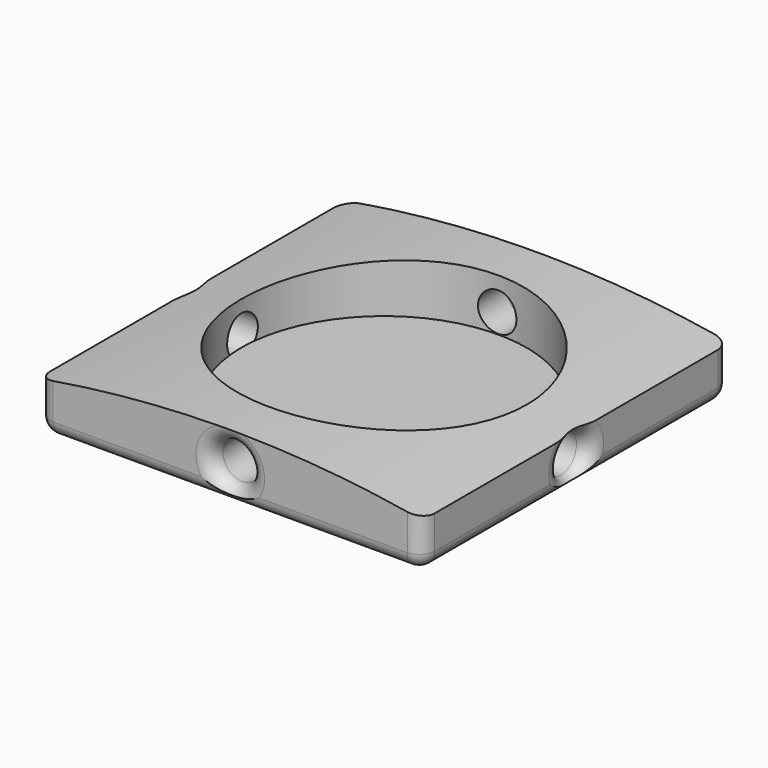
from build123d import *

# Parameters (mm, degrees)
F0_R         = 2.54
F1_DEPTH     = 25.4
F2_R         = 2.5365962647
F3_DEPTH     = 60.706
F4_R         = 18.8716899986
F5_DEPTH     = 14.478
F6_DEPTH     = 1.778
F7_T1_DEPTH  = 46.7340686292
F7_T3_DEPTH  = 46.7340686292
F7_T5_DEPTH  = 9.4612519522
F7_S9_W      = 2.2367022539
F7_S9_H      = 2.2367022539
F7_T10_DEPTH = 2.236702254
F7_S15_W     = 2.2367022539
F7_S15_H     = 2.2367022539
F7_T16_DEPTH = 2.236702254
F7_S21_W     = 2.2367022539
F7_S21_H     = 2.2367022539
F7_T22_DEPTH = 2.236702254
F7_S27_W     = 2.2367022539
F7_S27_H     = 2.2367022539
F7_T28_DEPTH = 2.236702254


# Not quite as in the source:
# - a fillet or chamfer that OpenCascade refuses, or shapes differently, is made with other operations: its cross-section is extruded or revolved along the edge and cut away or added


with BuildPart() as f1:
    # F0 (on Front) → F1 (new body, symmetric)
    with BuildSketch(Plane.XZ):
        with BuildLine():
            Line((25.4, 14.5918969065), (25.4, 21.0037002322))
            ThreePointArc((25.4, 21.0037002322), (0, 23.2693725585), (-25.4, 21.0037002322))
            Line((-25.4, 21.0037002322), (-25.4, 14.5918969065))
            Line((-25.4, 14.5918969065), (25.4, 14.5918969065))
        make_face()
        with Locations((0, 18.9952347428)):
            Circle(F0_R, mode=Mode.SUBTRACT)
    extrude(amount=F1_DEPTH, both=True)

    # F2 (on face) → F3 (cut)
    with BuildSketch(Plane.YZ.offset(25.4)):
        with Locations((0, 17.843645066)):
            Circle(F2_R)
    extrude(amount=-F3_DEPTH, mode=Mode.SUBTRACT)

    # F4 (on face) → F5 (cut)
    with BuildSketch(Plane(origin=(0, 0, 14.5918969065), x_dir=(1, 0, 0), z_dir=(0, 0, -1))):
        Circle(F4_R)
    extrude(amount=-F5_DEPTH, mode=Mode.SUBTRACT)

    # F4 (on face) → F6 (join)
    with BuildSketch(Plane(origin=(0, 0, 14.5918969065), x_dir=(1, 0, 0), z_dir=(0, 0, -1))):
        Circle(F4_R)
    extrude(amount=-F6_DEPTH)

    # F7: fillet of radius 2.032 on 12 edges, made by hand

    # F7_s2 → F7_t1 (cut)
    with BuildSketch(Plane.XZ.offset(-23.3670343146)):
        with BuildLine():
            ThreePointArc((-25.4004, 16.6248625919), (-24.8048409794, 15.1870559271), (-23.3670343146, 14.5914969065))
            Line((-23.3670343146, 14.5914969065), (-23.3670343146, 14.388160338))
            ThreePointArc((-23.3670343146, 14.388160338), (-24.3835171573, 14.388560338), (-25.4, 14.388560338))
            Line((-25.4, 14.388560338), (-25.6033365685, 14.5918969065))
            ThreePointArc((-25.6033365685, 14.5918969065), (-25.6033365685, 15.6083797492), (-25.6037365685, 16.6248625919))
            Line((-25.6037365685, 16.6248625919), (-25.4004, 16.6248625919))
        make_face()
        with BuildLine():
            ThreePointArc((25.4004, 16.6248625919), (24.8048409794, 15.1870559271), (23.3670343146, 14.5914969065))
            Line((23.3670343146, 14.5914969065), (23.3670343146, 14.388160338))
            ThreePointArc((23.3670343146, 14.388160338), (24.3835171573, 14.388560338), (25.4, 14.388560338))
            Line((25.4, 14.388560338), (25.6033365685, 14.5918969065))
            ThreePointArc((25.6033365685, 14.5918969065), (25.6033365685, 15.6083797492), (25.6037365685, 16.6248625919))
            Line((25.6037365685, 16.6248625919), (25.4004, 16.6248625919))
        make_face()
    extrude(amount=F7_T1_DEPTH, mode=Mode.SUBTRACT)

    # F7_s4 → F7_t3 (cut)
    with BuildSketch(Plane.YZ.offset(-23.3670343146)):
        with BuildLine():
            ThreePointArc((23.3670343146, 14.5914969065), (24.8048409794, 15.1870559271), (25.4004, 16.6248625919))
            Line((25.4004, 16.6248625919), (25.6037365685, 16.6248625919))
            ThreePointArc((25.6037365685, 16.6248625919), (25.6033365685, 15.6083797492), (25.6033365685, 14.5918969065))
            Line((25.6033365685, 14.5918969065), (25.4, 14.388560338))
            ThreePointArc((25.4, 14.388560338), (24.3835171573, 14.388560338), (23.3670343146, 14.388160338))
            Line((23.3670343146, 14.388160338), (23.3670343146, 14.5914969065))
        make_face()
        with BuildLine():
            ThreePointArc((-25.4004, 16.6248625919), (-24.8048409794, 15.1870559271), (-23.3670343146, 14.5914969065))
            Line((-23.3670343146, 14.5914969065), (-23.3670343146, 14.388160338))
            ThreePointArc((-23.3670343146, 14.388160338), (-24.3835171573, 14.388560338), (-25.4, 14.388560338))
            Line((-25.4, 14.388560338), (-25.6033365685, 14.5918969065))
            ThreePointArc((-25.6033365685, 14.5918969065), (-25.6033365685, 15.6083797492), (-25.6037365685, 16.6248625919))
            Line((-25.6037365685, 16.6248625919), (-25.4004, 16.6248625919))
        make_face()
    extrude(amount=F7_T3_DEPTH, mode=Mode.SUBTRACT)

    # F7_s6 → F7_t5 (cut)
    with BuildSketch(Plane.XY.offset(16.6248625919)):
        with BuildLine():
            ThreePointArc((-25.4004, 23.3670343146), (-24.8048409794, 24.8048409794), (-23.3670343146, 25.4004))
            Line((-23.3670343146, 25.4004), (-23.3670343146, 25.6037365685))
            ThreePointArc((-23.3670343146, 25.6037365685), (-24.3835171573, 25.6033365685), (-25.4, 25.6033365685))
            Line((-25.4, 25.6033365685), (-25.6033365685, 25.4))
            ThreePointArc((-25.6033365685, 25.4), (-25.6033365685, 24.3835171573), (-25.6037365685, 23.3670343146))
            Line((-25.6037365685, 23.3670343146), (-25.4004, 23.3670343146))
        make_face()
        with BuildLine():
            ThreePointArc((-25.4004, -23.3670343146), (-24.8048409794, -24.8048409794), (-23.3670343146, -25.4004))
            Line((-23.3670343146, -25.4004), (-23.3670343146, -25.6037365685))
            ThreePointArc((-23.3670343146, -25.6037365685), (-24.3835171573, -25.6033365685), (-25.4, -25.6033365685))
            Line((-25.4, -25.6033365685), (-25.6033365685, -25.4))
            ThreePointArc((-25.6033365685, -25.4), (-25.6033365685, -24.3835171573), (-25.6037365685, -23.3670343146))
            Line((-25.6037365685, -23.3670343146), (-25.4004, -23.3670343146))
        make_face()
        with BuildLine():
            ThreePointArc((25.4004, -23.3670343146), (24.8048409794, -24.8048409794), (23.3670343146, -25.4004))
            Line((23.3670343146, -25.4004), (23.3670343146, -25.6037365685))
            ThreePointArc((23.3670343146, -25.6037365685), (24.3835171573, -25.6033365685), (25.4, -25.6033365685))
            Line((25.4, -25.6033365685), (25.6033365685, -25.4))
            ThreePointArc((25.6033365685, -25.4), (25.6033365685, -24.3835171573), (25.6037365685, -23.3670343146))
            Line((25.6037365685, -23.3670343146), (25.4004, -23.3670343146))
        make_face()
        with BuildLine():
            ThreePointArc((25.4004, 23.3670343146), (24.8048409794, 24.8048409794), (23.3670343146, 25.4004))
            Line((23.3670343146, 25.4004), (23.3670343146, 25.6037365685))
            ThreePointArc((23.3670343146, 25.6037365685), (24.3835171573, 25.6033365685), (25.4, 25.6033365685))
            Line((25.4, 25.6033365685), (25.6033365685, 25.4))
            ThreePointArc((25.6033365685, 25.4), (25.6033365685, 24.3835171573), (25.6037365685, 23.3670343146))
            Line((25.6037365685, 23.3670343146), (25.4004, 23.3670343146))
        make_face()
    extrude(amount=F7_T5_DEPTH, mode=Mode.SUBTRACT)


with BuildPart() as f7_tool8:
    # F7_s9 → F7_t10 (new body)
    with BuildSketch(Plane.YZ.offset(-23.3670343146)):
        with Locations((24.4853854416, 15.506511465)):
            Rectangle(F7_S9_W, F7_S9_H)
    extrude(amount=-F7_T10_DEPTH)

    # F7_s11 → F7_t12 (revolve, cut)
    with BuildSketch(Plane(origin=(-23.3670343146, 23.3670343146, 16.6248625919), x_dir=(0, -0.7071067812, 0.7071067812), z_dir=(0, -0.7071067812, -0.7071067812))):
        with BuildLine():
            ThreePointArc((0, -2.0333656854), (2.0333656854, 0), (0, 2.0333656854))
            Line((0, 2.0333656854), (0, -2.0333656854))
        make_face()
    revolve(axis=Axis((-23.3670343146, 23.3670343146, 16.6248625919), (-1, 0, 0)), mode=Mode.SUBTRACT)


with BuildPart() as f1_1:
    add(f1.part)

    # F7_t7: cut F7_tool8
    add(f7_tool8.part, mode=Mode.SUBTRACT)


with BuildPart() as f7_tool14:
    # F7_s15 → F7_t16 (new body)
    with BuildSketch(Plane.YZ.offset(-23.3670343146)):
        with Locations((-24.4853854416, 15.506511465)):
            Rectangle(F7_S15_W, F7_S15_H)
    extrude(amount=-F7_T16_DEPTH)

    # F7_s17 → F7_t18 (revolve, cut)
    with BuildSketch(Plane(origin=(-23.3670343146, -23.3670343146, 16.6248625919), x_dir=(0, 0.7071067812, 0.7071067812), z_dir=(0, -0.7071067812, 0.7071067812))):
        with BuildLine():
            ThreePointArc((0, -2.0333656854), (2.0333656854, 0), (0, 2.0333656854))
            Line((0, 2.0333656854), (0, -2.0333656854))
        make_face()
    revolve(axis=Axis((-23.3670343146, -23.3670343146, 16.6248625919), (-1, 0, 0)), mode=Mode.SUBTRACT)


with BuildPart() as f1_2:
    add(f1_1.part)

    # F7_t13: cut F7_tool14
    add(f7_tool14.part, mode=Mode.SUBTRACT)


with BuildPart() as f7_tool20:
    # F7_s21 → F7_t22 (new body)
    with BuildSketch(Plane.XY.offset(16.6248625919)):
        with Locations((24.4853854416, 24.4853854416)):
            Rectangle(F7_S21_W, F7_S21_H)
    extrude(amount=-F7_T22_DEPTH)

    # F7_s23 → F7_t24 (revolve, cut)
    with BuildSketch(Plane(origin=(23.3670343146, 23.3670343146, 16.6248625919), x_dir=(-0.7071067812, -0.7071067812, 0), z_dir=(0.7071067812, -0.7071067812, 0))):
        with BuildLine():
            ThreePointArc((0, -2.0333656854), (2.0333656854, 0), (0, 2.0333656854))
            Line((0, 2.0333656854), (0, -2.0333656854))
        make_face()
    revolve(axis=Axis((23.3670343146, 23.3670343146, 16.6248625919), (0, 0, -1)), mode=Mode.SUBTRACT)


with BuildPart() as f1_3:
    add(f1_2.part)

    # F7_t19: cut F7_tool20
    add(f7_tool20.part, mode=Mode.SUBTRACT)


with BuildPart() as f7_tool26:
    # F7_s27 → F7_t28 (new body)
    with BuildSketch(Plane.XZ.offset(23.3670343146)):
        with Locations((24.4853854416, 15.506511465)):
            Rectangle(F7_S27_W, F7_S27_H)
    extrude(amount=F7_T28_DEPTH)

    # F7_s29 → F7_t30 (revolve, cut)
    with BuildSketch(Plane(origin=(23.3670343146, -23.3670343146, 16.6248625919), x_dir=(-0.7071067812, 0, 0.7071067812), z_dir=(0.7071067812, 0, 0.7071067812))):
        with BuildLine():
            ThreePointArc((0, -2.0333656854), (2.0333656854, 0), (0, 2.0333656854))
            Line((0, 2.0333656854), (0, -2.0333656854))
        make_face()
    revolve(axis=Axis((23.3670343146, -23.3670343146, 16.6248625919), (0, -1, 0)), mode=Mode.SUBTRACT)


with BuildPart() as f1_4:
    add(f1_3.part)

    # F7_t25: cut F7_tool26
    add(f7_tool26.part, mode=Mode.SUBTRACT)

    # F7_s31 → F7_t32 (revolve, cut)
    with BuildSketch(Plane.XY.offset(18.9952347428)):
        with BuildLine():
            ThreePointArc((2.5396, 23.3670343146), (3.1351590206, 24.8048409794), (4.5729656854, 25.4004))
            Line((4.5729656854, 25.4004), (4.5729656854, 25.6037365685))
            ThreePointArc((4.5729656854, 25.6037365685), (3.5564828427, 25.6033365685), (2.54, 25.6033365685))
            Line((2.54, 25.6033365685), (2.3366634315, 25.4))
            ThreePointArc((2.3366634315, 25.4), (2.3366634315, 24.3835171573), (2.3362634315, 23.3670343146))
            Line((2.3362634315, 23.3670343146), (2.5396, 23.3670343146))
        make_face()
    revolve(axis=Axis((0, 25.4, 18.9952347428), (0, -1, 0)), mode=Mode.SUBTRACT)

    # F7_s33 → F7_t34 (revolve, cut)
    with BuildSketch(Plane.XY.offset(17.843645066)):
        with BuildLine():
            ThreePointArc((23.3670343146, 2.5361962647), (24.8048409794, 3.1317552853), (25.4004, 4.5695619501))
            Line((25.4004, 4.5695619501), (25.6037365685, 4.5695619501))
            ThreePointArc((25.6037365685, 4.5695619501), (25.6033365685, 3.5530791074), (25.6033365685, 2.5365962647))
            Line((25.6033365685, 2.5365962647), (25.4, 2.3332596961))
            ThreePointArc((25.4, 2.3332596961), (24.3835171573, 2.3332596961), (23.3670343146, 2.3328596961))
            Line((23.3670343146, 2.3328596961), (23.3670343146, 2.5361962647))
        make_face()
    revolve(axis=Axis((25.4, 0, 17.843645066), (1, 0, 0)), mode=Mode.SUBTRACT)

    # F7_s35 → F7_t36 (revolve, cut)
    with BuildSketch(Plane.XY.offset(18.9952347428)):
        with BuildLine():
            ThreePointArc((2.5396, -23.3670343146), (3.1351590206, -24.8048409794), (4.5729656854, -25.4004))
            Line((4.5729656854, -25.4004), (4.5729656854, -25.6037365685))
            ThreePointArc((4.5729656854, -25.6037365685), (3.5564828427, -25.6033365685), (2.54, -25.6033365685))
            Line((2.54, -25.6033365685), (2.3366634315, -25.4))
            ThreePointArc((2.3366634315, -25.4), (2.3366634315, -24.3835171573), (2.3362634315, -23.3670343146))
            Line((2.3362634315, -23.3670343146), (2.5396, -23.3670343146))
        make_face()
    revolve(axis=Axis((0, -25.4, 18.9952347428), (0, -1, 0)), mode=Mode.SUBTRACT)

    # F7_s37 → F7_t38 (revolve, cut)
    with BuildSketch(Plane.XY.offset(17.843645066)):
        with BuildLine():
            ThreePointArc((-25.4004, 4.5695619501), (-24.8048409794, 3.1317552853), (-23.3670343146, 2.5361962647))
            Line((-23.3670343146, 2.5361962647), (-23.3670343146, 2.3328596961))
            ThreePointArc((-23.3670343146, 2.3328596961), (-24.3835171573, 2.3332596961), (-25.4, 2.3332596961))
            Line((-25.4, 2.3332596961), (-25.6033365685, 2.5365962647))
            ThreePointArc((-25.6033365685, 2.5365962647), (-25.6033365685, 3.5530791074), (-25.6037365685, 4.5695619501))
            Line((-25.6037365685, 4.5695619501), (-25.4004, 4.5695619501))
        make_face()
    revolve(axis=Axis((-25.4, 0, 17.843645066), (1, 0, 0)), mode=Mode.SUBTRACT)


solid = f1_4.part
